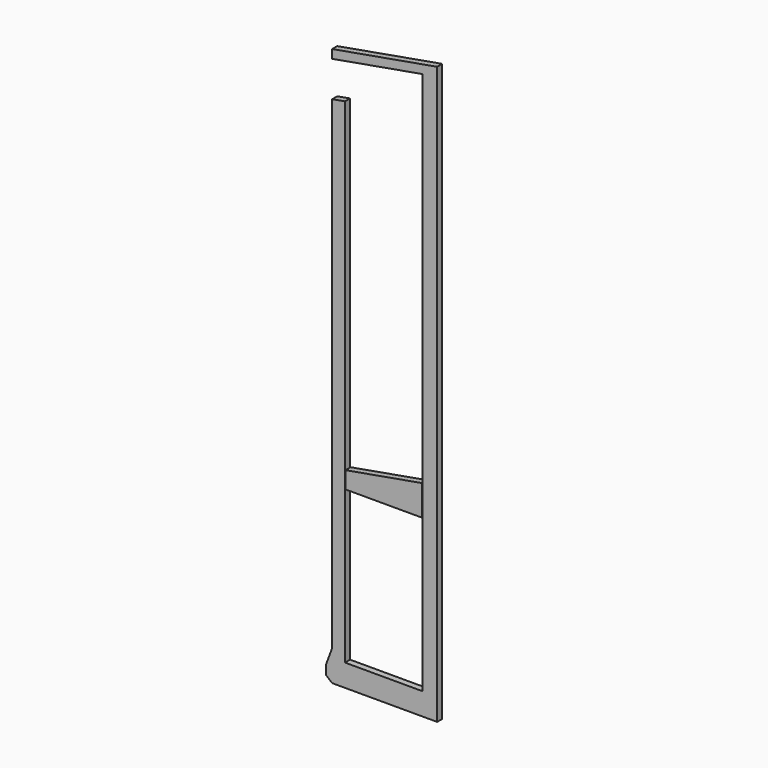
from build123d import *

# Parameters (mm, degrees)
F1_DEPTH = 3
F2_DEPTH = 3


# Not quite as in the source:
# - a feature names something its author has since deleted; it is built from what else it names


with BuildPart() as f1:
    # F0 (on Front) → F1 (new body)
    with BuildSketch(Plane.XZ):
        Polygon((-43.1878868615, -160.5870006293), (-43.1878868615, -168.5870006293), (-7.25, -168.5870006293), (-7.25, -154.250181546), align=None)
    extrude(amount=F1_DEPTH)


with BuildPart() as f2:
    # F0 (on Front) → F2 (new body)
    with BuildSketch(Plane.XZ):
        Polygon((-49.5, -251), (0, -251), (0, 0), (0, 20.8162455437), (-49.5, 12.0880599986), (-49.5, 8.026353551), (-7, 15.5202502312), (-7, -1.234288865), (-7, -240.5024516791), (-43.4378868615, -240.5024516791), (-43.4378868615, -7.6592714386), (-49.5, -8.7281855451), (-49.5, -236.5), (-52.5, -244.5), (-52.5, -248.5), align=None)
    extrude(amount=F2_DEPTH)


solid = Compound([f1.part, f2.part])
